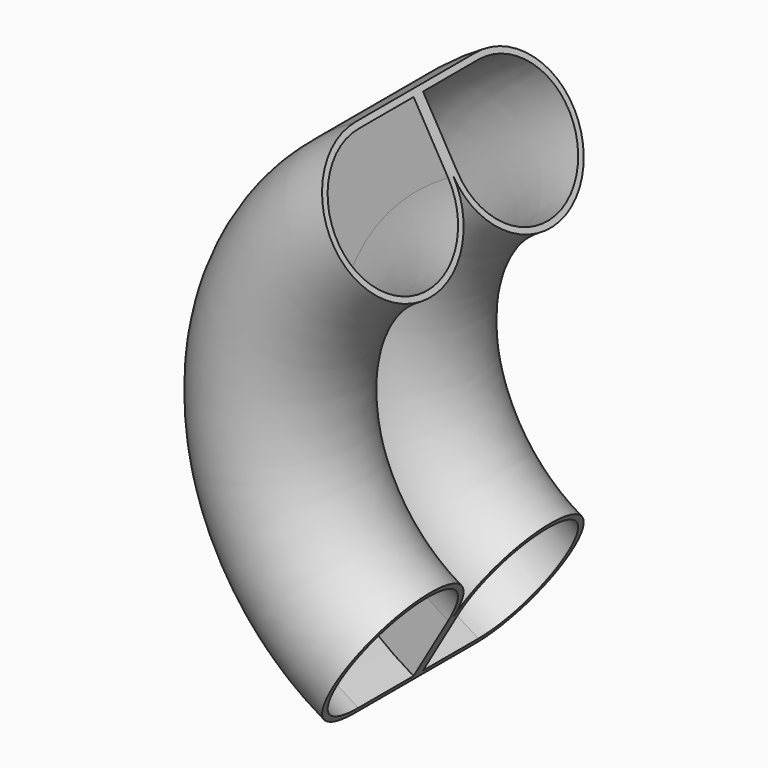
from build123d import *

# Parameters (mm, degrees)
F1_ANGLE_BACK = 60
F1_ANGLE      = 120
F2_T          = -5


with BuildPart() as f1:
    # F0 (on Top) → F1 (revolve)
    with BuildSketch(Plane.XY, mode=Mode.PRIVATE) as f1_sk:
        with BuildLine():
            Line((-12.6999996577, 50.8), (-76.2, 50.8))
            Line((-76.2, 50.8), (-76.2, -12.6999997152))
            ThreePointArc((-76.2, -12.6999997152), (-57.6012803836, 32.2012808271), (-12.6999996577, 50.8))
        make_face()
        with BuildLine():
            ThreePointArc((50.8, -12.7), (32.2012807264, 32.2012804843), (-12.6999996577, 50.8))
            ThreePointArc((-12.6999996577, 50.8), (-57.6012803836, 32.2012808271), (-76.2, -12.6999997152))
            ThreePointArc((-76.2, -12.6999997152), (-12.7000001424, -76.2), (50.8, -12.7))
        make_face()
    revolve(f1_sk.sketch.rotate(Axis((177.8, -25.4, 0), (0, -1, 0)), -F1_ANGLE_BACK), axis=Axis((177.8, -25.4, 0), (0, -1, 0)), revolution_arc=F1_ANGLE)

    # F2
    f2_openings = [f1.faces().sort_by_distance(p)[0] for p in [
        (80.973313, -9.546627, 167.708741),
        (80.973313, -9.546627, -167.708741),
    ]]
    offset(amount=F2_T, openings=f2_openings, kind=Kind.INTERSECTION)

    # F4: F1 across plane


with BuildPart() as f1_1:
    add(f1.part)
    add(f1.part.mirror(Plane(origin=(-7.2496055577, 50.8, 0), x_dir=(-1, 0, 0), z_dir=(0, 1, 0))))


solid = f1_1.part
